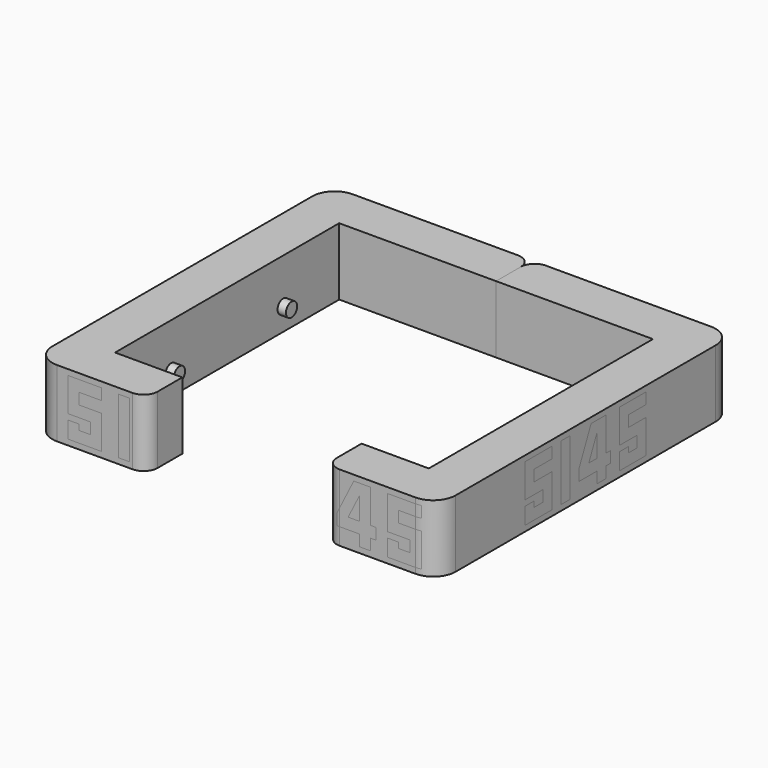
from build123d import *

# Parameters (mm, degrees)
F1_DEPTH       = 15.24
F2_R           = 1.5875
F3_DEPTH       = 1.905
F5_DEPTH       = 15.24
F6_R           = 1.5875
F7_DEPTH       = 1.905
F8_W           = 2.54
F8_H           = 12.7
F9_DEPTH       = 0.79375
F11_DEPTH      = 0.79375
F12_W          = 2.54
F12_H          = 12.7
F13_DEPTH      = 0.79375
F14_W          = 2.54
F14_H          = 12.7
F15_DEPTH      = 0.79375
F16_W          = 2.54
F16_H          = 12.7
F17_DEPTH      = 0.79375
F19_DEPTH      = 0.79375
F20_R          = 5.08
F21_T1_DEPTH   = 40.64
F22_T1_DEPTH   = 31.115
F22_2_T1_DEPTH = 31.115
F23_DEPTH      = 0.79375
F24_DEPTH      = 0.79375
F25_DEPTH      = 0.79375
F26_DEPTH      = 0.79375
F28_DEPTH      = 25.4
F30_DEPTH      = 25.4
F32_DEPTH      = 25.4


# Not quite as in the source:
# - a fillet or chamfer that OpenCascade refuses, or shapes differently, is made with other operations: its cross-section is extruded or revolved along the edge and cut away or added


with BuildPart() as f1:
    # F0 (on Top) → F1 (new body)
    with BuildSketch(Plane.XY):
        Polygon((0, 38.8312135783), (0, 28.6712135783), (35.56, 28.6712135783), (35.56, -34.8287864217), (20.32, -34.8287864217), (20.32, -44.9887864217), (45.72, -44.9887864217), (45.72, 38.8312135783), align=None)
    extrude(amount=F1_DEPTH)

    # F2 (on face) → F3 (join)
    with BuildSketch(Plane(origin=(35.56, 0, 0), x_dir=(0, -1, 0), z_dir=(-1, 0, 0))):
        with Locations((-12.7962135783, 5.08)):
            Circle(F2_R)
        with Locations((18.9537864217, 5.08)):
            Circle(F2_R)
    extrude(amount=F3_DEPTH)

    # F8 (on face) → F9 (cut)
    with BuildSketch(Plane.YZ.offset(45.72)):
        Polygon((-12.6037864217, 11.43), (-12.6037864217, 13.97), (-20.2237864217, 13.97), (-20.2237864217, 6.35), (-15.1437864217, 6.35), (-15.1437864217, 3.81), (-17.6837864217, 3.81), (-17.6837864217, 5.08), (-20.2237864217, 5.08), (-20.2237864217, 1.27), (-12.6037864217, 1.27), (-12.6037864217, 8.89), (-17.6837864217, 8.89), (-17.6837864217, 11.43), align=None)
        with Locations((-8.7937864217, 7.62)):
            Rectangle(F8_W, F8_H)
        Polygon((2.6362135783, 13.97), (-1.5439947518, 13.97), (-4.9837864217, 6.35), (-4.9837864217, 3.81), (0.0962135783, 3.81), (0.0962135783, 1.27), (2.6362135783, 1.27), (2.6362135783, 3.81), (3.9062135783, 3.81), (3.9062135783, 6.35), (2.6362135783, 6.35), align=None)
        Polygon((0.0962135783, 11.43), (0.0962135783, 6.35), (-2.1969808683, 6.35), align=None, mode=Mode.SUBTRACT)
        Polygon((14.0662135783, 11.43), (14.0662135783, 13.97), (6.4462135783, 13.97), (6.4462135783, 6.35), (11.5262135783, 6.35), (11.5262135783, 3.81), (8.9862135783, 3.81), (8.9862135783, 5.08), (6.4462135783, 5.08), (6.4462135783, 1.27), (14.0662135783, 1.27), (14.0662135783, 8.89), (8.9862135783, 8.89), (8.9862135783, 11.43), align=None)
    extrude(amount=-F9_DEPTH, mode=Mode.SUBTRACT)

    # F10 (on face) → F11 (cut)
    with BuildSketch(Plane.XZ.offset(44.9887864217)):
        Polygon((26.67, 13.97), (22.86, 6.35), (22.86, 3.81), (27.94, 3.81), (27.94, 1.27), (30.48, 1.27), (30.48, 3.81), (31.75, 3.81), (31.75, 6.35), (30.48, 6.35), (30.48, 13.97), align=None)
        Polygon((27.94, 11.43), (27.94, 6.35), (25.4, 6.35), align=None, mode=Mode.SUBTRACT)
        Polygon((41.91, 11.43), (41.91, 13.97), (34.29, 13.97), (34.29, 6.35), (39.37, 6.35), (39.37, 3.81), (36.83, 3.81), (36.83, 5.08), (34.29, 5.08), (34.29, 1.27), (41.91, 1.27), (41.91, 8.89), (36.83, 8.89), (36.83, 11.43), align=None)
    extrude(amount=-F11_DEPTH, mode=Mode.SUBTRACT)

    # F16 (on face) → F17 (cut)
    with BuildSketch(Plane(origin=(0, 38.8312135783, 0), x_dir=(-1, 0, 0), z_dir=(0, 1, 0))):
        Polygon((-8.89, 11.43), (-8.89, 13.97), (-16.51, 13.97), (-16.51, 6.35), (-11.43, 6.35), (-11.43, 3.81), (-13.97, 3.81), (-13.97, 5.08), (-16.51, 5.08), (-16.51, 1.27), (-8.89, 1.27), (-8.89, 8.89), (-13.97, 8.89), (-13.97, 11.43), align=None)
        with Locations((-5.08, 7.62)):
            Rectangle(F16_W, F16_H)
    extrude(amount=-F17_DEPTH, mode=Mode.SUBTRACT)

    # F21: fillet of radius 5.08 on 2 edges, made by hand

    # F21_s2 → F21_t1 (cut)
    with BuildSketch(Plane.XY.offset(-12.7)):
        with BuildLine():
            ThreePointArc((45.72, -39.9087864217), (44.2321024484, -43.5008888701), (40.64, -44.9887864217))
            Line((40.64, -44.9887864217), (45.72, -44.9887864217))
            Line((45.72, -44.9887864217), (45.72, -39.9087864217))
        make_face()
        with BuildLine():
            ThreePointArc((40.64, 38.8312135783), (44.2321024484, 37.3433160267), (45.72, 33.7512135783))
            Line((45.72, 33.7512135783), (45.72, 38.8312135783))
            Line((45.72, 38.8312135783), (40.64, 38.8312135783))
        make_face()
    extrude(amount=F21_T1_DEPTH, mode=Mode.SUBTRACT)

    # F22: fillet of radius 3.175 on 2 edges, made by hand

    # F22_s2 → F22_t1 (cut)
    with BuildSketch(Plane.XY.offset(-7.9375)):
        with BuildLine():
            ThreePointArc((23.495, -44.9887864217), (21.2499359697, -44.058850452), (20.32, -41.8137864217))
            Line((20.32, -41.8137864217), (20.32, -44.9887864217))
            Line((20.32, -44.9887864217), (23.495, -44.9887864217))
        make_face()
        with BuildLine():
            ThreePointArc((0, 35.6562135783), (0.9299359697, 37.9012776086), (3.175, 38.8312135783))
            Line((3.175, 38.8312135783), (0, 38.8312135783))
            Line((0, 38.8312135783), (0, 35.6562135783))
        make_face()
    extrude(amount=F22_T1_DEPTH, mode=Mode.SUBTRACT)


with BuildPart() as f5:
    # F4 (on Top) → F5 (new body)
    with BuildSketch(Plane.XY):
        Polygon((-35.56, 28.6712135783), (0, 28.6712135783), (0, 38.8312135783), (-45.72, 38.8312135783), (-45.72, -44.9887864217), (-20.32, -44.9887864217), (-20.32, -34.8287864217), (-35.56, -34.8287864217), align=None)
    extrude(amount=F5_DEPTH)

    # F6 (on face) → F7 (join)
    with BuildSketch(Plane.YZ.offset(-35.56)):
        with Locations((12.7962135783, 5.08)):
            Circle(F6_R)
        with Locations((-18.9537864217, 5.08)):
            Circle(F6_R)
    extrude(amount=F7_DEPTH)

    # F12 (on face) → F13 (cut)
    with BuildSketch(Plane.XZ.offset(44.9887864217)):
        Polygon((-30.48, 11.43), (-30.48, 13.97), (-38.1, 13.97), (-38.1, 6.35), (-33.02, 6.35), (-33.02, 3.81), (-35.56, 3.81), (-35.56, 5.08), (-38.1, 5.08), (-38.1, 1.27), (-30.48, 1.27), (-30.48, 8.89), (-35.56, 8.89), (-35.56, 11.43), align=None)
        with Locations((-25.4, 7.62)):
            Rectangle(F12_W, F12_H)
    extrude(amount=-F13_DEPTH, mode=Mode.SUBTRACT)

    # F14 (on face) → F15 (cut)
    with BuildSketch(Plane(origin=(-45.72, 0, 0), x_dir=(0, -1, 0), z_dir=(-1, 0, 0))):
        Polygon((-6.4462135783, 11.43), (-6.4462135783, 13.97), (-14.0662135783, 13.97), (-14.0662135783, 6.35), (-8.9862135783, 6.35), (-8.9862135783, 3.81), (-11.5262135783, 3.81), (-11.5262135783, 5.08), (-14.0662135783, 5.08), (-14.0662135783, 1.27), (-6.4462135783, 1.27), (-6.4462135783, 8.89), (-11.5262135783, 8.89), (-11.5262135783, 11.43), align=None)
        with Locations((-2.6362135783, 7.62)):
            Rectangle(F14_W, F14_H)
        Polygon((8.7937864217, 13.97), (4.9837864217, 13.97), (1.1737864217, 6.35), (1.1737864217, 3.81), (6.2537864217, 3.81), (6.2537864217, 1.27), (8.7937864217, 1.27), (8.7937864217, 3.81), (10.0637864217, 3.81), (10.0637864217, 6.35), (8.7937864217, 6.35), align=None)
        Polygon((6.2537864217, 11.43), (6.2537864217, 6.35), (3.7137864217, 6.35), align=None, mode=Mode.SUBTRACT)
        Polygon((20.2237864217, 11.43), (20.2237864217, 13.97), (12.6037864217, 13.97), (12.6037864217, 6.35), (17.6837864217, 6.35), (17.6837864217, 3.81), (15.1437864217, 3.81), (15.1437864217, 5.08), (12.6037864217, 5.08), (12.6037864217, 1.27), (20.2237864217, 1.27), (20.2237864217, 8.89), (15.1437864217, 8.89), (15.1437864217, 11.43), align=None)
    extrude(amount=-F15_DEPTH, mode=Mode.SUBTRACT)

    # F18 (on face) → F19 (cut)
    with BuildSketch(Plane(origin=(0, 38.8312135783, 0), x_dir=(-1, 0, 0), z_dir=(0, 1, 0))):
        Polygon((6.35, 13.97), (2.54, 6.35), (2.54, 3.81), (7.62, 3.81), (7.62, 1.27), (10.16, 1.27), (10.16, 3.81), (11.43, 3.81), (11.43, 6.35), (10.16, 6.35), (10.16, 13.97), align=None)
        Polygon((7.62, 11.43), (7.62, 6.35), (5.08, 6.35), align=None, mode=Mode.SUBTRACT)
        Polygon((21.59, 11.43), (21.59, 13.97), (13.97, 13.97), (13.97, 6.35), (19.05, 6.35), (19.05, 3.81), (16.51, 3.81), (16.51, 5.08), (13.97, 5.08), (13.97, 1.27), (21.59, 1.27), (21.59, 8.89), (16.51, 8.89), (16.51, 11.43), align=None)
    extrude(amount=-F19_DEPTH, mode=Mode.SUBTRACT)

    # F20
    f20_edges = [f5.edges().sort_by_distance(p)[0] for p in [
        (-45.72, 38.831214, 7.62),
        (-45.72, -44.988786, 7.62),
    ]]
    fillet(f20_edges, radius=F20_R)

    # F22#2: fillet of radius 3.175 on 2 edges, made by hand

    # F22_2_s2 → F22_2_t1 (cut)
    with BuildSketch(Plane.XY.offset(-7.9375)):
        with BuildLine():
            ThreePointArc((-23.495, -44.9887864217), (-21.2499359697, -44.058850452), (-20.32, -41.8137864217))
            Line((-20.32, -41.8137864217), (-20.32, -44.9887864217))
            Line((-20.32, -44.9887864217), (-23.495, -44.9887864217))
        make_face()
        with BuildLine():
            ThreePointArc((-3.175, 38.8312135783), (-0.9299359697, 37.9012776086), (0, 35.6562135783))
            Line((0, 35.6562135783), (0, 38.8312135783))
            Line((0, 38.8312135783), (-3.175, 38.8312135783))
        make_face()
    extrude(amount=F22_2_T1_DEPTH, mode=Mode.SUBTRACT)


with BuildPart() as f23:
    # F23 (new): a face of the model
    f23_faces = [f1.part.faces().sort_by_distance(p)[0] for p in [
        (24.9036570157, -44.1950364217, 10.0906714922),
    ]]
    extrude(f23_faces, amount=F23_DEPTH)

    # F29 (on face) → F30 (cut)
    with BuildSketch(Plane(origin=(0, 0, 3.81), x_dir=(1, 0, 0), z_dir=(0, 0, -1))):
        with BuildLine():
            ThreePointArc((22.86, 44.924638395), (23.1758840456, 44.9727087075), (23.495, 44.9887864217))
            Line((23.495, 44.9887864217), (22.86, 44.9887864217))
            Line((22.86, 44.9887864217), (22.86, 44.924638395))
        make_face()
    extrude(amount=-F30_DEPTH, mode=Mode.SUBTRACT)


with BuildPart() as f23b:
    # F23#2 (new): a face of the model
    f23_2_faces = [f1.part.faces().sort_by_distance(p)[0] for p in [
        (37.9895652174, -44.1950364217, 7.4819565217),
    ]]
    extrude(f23_2_faces, amount=F23_DEPTH)

    # F27 (on face) → F28 (cut)
    with BuildSketch(Plane(origin=(0, 0, 1.27), x_dir=(1, 0, 0), z_dir=(0, 0, -1))):
        with BuildLine():
            ThreePointArc((40.64, 44.9887864217), (41.2801018058, 44.9482972787), (41.91, 44.8274752714))
            Line((41.91, 44.8274752714), (41.91, 44.9887864217))
            Line((41.91, 44.9887864217), (40.64, 44.9887864217))
        make_face()
    extrude(amount=-F28_DEPTH, mode=Mode.SUBTRACT)


with BuildPart() as f23c:
    # F23#3 (new): a face of the model
    f23_3_faces = [f5.part.faces().sort_by_distance(p)[0] for p in [
        (-25.4, -44.1950364217, 7.62),
    ]]
    extrude(f23_3_faces, amount=F23_DEPTH)


with BuildPart() as f23d:
    # F23#4 (new): a face of the model
    f23_4_faces = [f5.part.faces().sort_by_distance(p)[0] for p in [
        (-34.4004347826, -44.1950364217, 7.4819565217),
    ]]
    extrude(f23_4_faces, amount=F23_DEPTH)


with BuildPart() as f24:
    # F24 (new): a face of the model
    f24_faces = [f5.part.faces().sort_by_distance(p)[0] for p in [
        (-44.92625, 10.3666483609, 7.4819565217),
    ]]
    extrude(f24_faces, amount=F24_DEPTH)


with BuildPart() as f24b:
    # F24#2 (new): a face of the model
    f24_2_faces = [f5.part.faces().sort_by_distance(p)[0] for p in [
        (-44.92625, 2.6362135783, 7.62),
    ]]
    extrude(f24_2_faces, amount=F24_DEPTH)


with BuildPart() as f24c:
    # F24#3 (new): a face of the model
    f24_3_faces = [f5.part.faces().sort_by_distance(p)[0] for p in [
        (-44.92625, -9.4287864217, 3.9650232563),
    ]]
    extrude(f24_3_faces, amount=F24_DEPTH)


with BuildPart() as f24d:
    # F24#4 (new): a face of the model
    f24_4_faces = [f5.part.faces().sort_by_distance(p)[0] for p in [
        (-44.92625, -16.3033516391, 7.4819565217),
    ]]
    extrude(f24_4_faces, amount=F24_DEPTH)


with BuildPart() as f25:
    # F25 (new): a face of the model
    f25_faces = [f1.part.faces().sort_by_distance(p)[0] for p in [
        (12.8104347826, 38.0374635783, 7.4819565217),
    ]]
    extrude(f25_faces, amount=F25_DEPTH)


with BuildPart() as f25b:
    # F25#2 (new): a face of the model
    f25_2_faces = [f1.part.faces().sort_by_distance(p)[0] for p in [
        (5.08, 38.0374635783, 7.62),
    ]]
    extrude(f25_2_faces, amount=F25_DEPTH)


with BuildPart() as f25c:
    # F25#3 (new): a face of the model
    f25_3_faces = [f5.part.faces().sort_by_distance(p)[0] for p in [
        (-4.5836570157, 38.0374635783, 10.0906714922),
    ]]
    extrude(f25_3_faces, amount=F25_DEPTH)

    # F31 (on face) → F32 (cut)
    with BuildSketch(Plane(origin=(0, 0, 3.81), x_dir=(1, 0, 0), z_dir=(0, 0, -1))):
        with BuildLine():
            ThreePointArc((-2.54, -38.7670655516), (-2.8558840456, -38.8151358641), (-3.175, -38.8312135783))
            Line((-3.175, -38.8312135783), (-2.54, -38.8312135783))
            Line((-2.54, -38.8312135783), (-2.54, -38.7670655516))
        make_face()
    extrude(amount=-F32_DEPTH, mode=Mode.SUBTRACT)


with BuildPart() as f25d:
    # F25#4 (new): a face of the model
    f25_4_faces = [f5.part.faces().sort_by_distance(p)[0] for p in [
        (-17.6695652174, 38.0374635783, 7.4819565217),
    ]]
    extrude(f25_4_faces, amount=F25_DEPTH)


with BuildPart() as f26:
    # F26 (new): a face of the model
    f26_faces = [f1.part.faces().sort_by_distance(p)[0] for p in [
        (44.92625, -16.5242212043, 7.4819565217),
    ]]
    extrude(f26_faces, amount=F26_DEPTH)


with BuildPart() as f26b:
    # F26#2 (new): a face of the model
    f26_2_faces = [f1.part.faces().sort_by_distance(p)[0] for p in [
        (44.92625, -8.7937864217, 7.62),
    ]]
    extrude(f26_2_faces, amount=F26_DEPTH)


with BuildPart() as f26c:
    # F26#3 (new): a face of the model
    f26_3_faces = [f1.part.faces().sort_by_distance(p)[0] for p in [
        (44.92625, 3.2712135783, 3.9650232563),
    ]]
    extrude(f26_3_faces, amount=F26_DEPTH)


with BuildPart() as f26d:
    # F26#4 (new): a face of the model
    f26_4_faces = [f1.part.faces().sort_by_distance(p)[0] for p in [
        (44.92625, 10.1457787957, 7.4819565217),
    ]]
    extrude(f26_4_faces, amount=F26_DEPTH)


solid = Compound([f1.part, f5.part, f23.part, f23b.part, f23c.part, f23d.part, f24.part, f24b.part, f24c.part, f24d.part, f25.part, f25b.part, f25c.part, f25d.part, f26.part, f26b.part, f26c.part, f26d.part])
